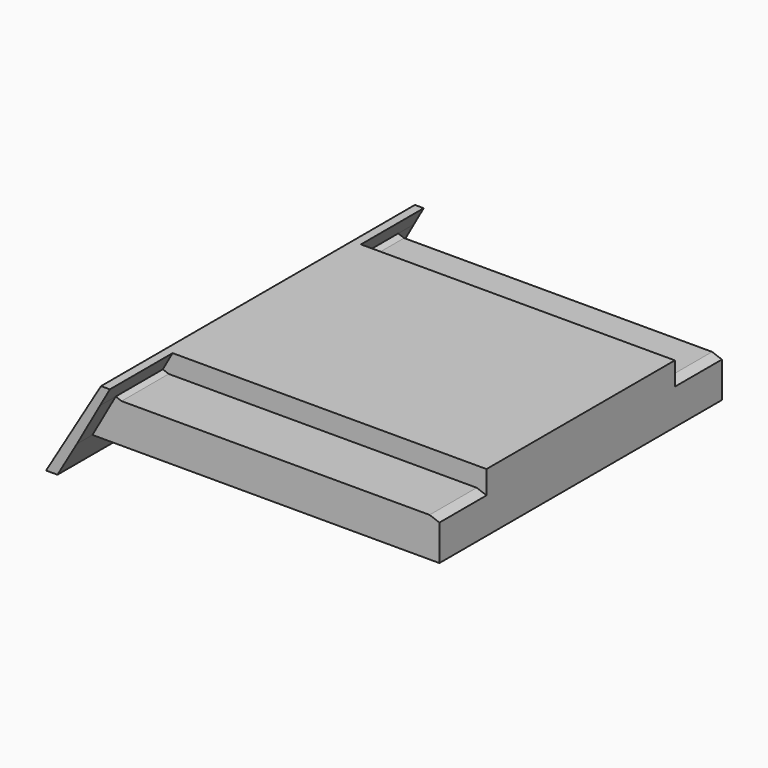
from build123d import *

# Parameters (mm, degrees)
F1_DEPTH  = 20
F3_DEPTH  = 4
F5_DEPTH  = 1
F7_DEPTH  = 20.001
F10_W     = 15
F10_H     = 9.1
F11_DEPTH = 1


# Not quite as in the source:
# - a pattern or mirror of a feature is missing from the dataset's text; its kind, count and spacing are read off the source's solid


with BuildPart() as f1:
    # F0 (on Front) → F1 (new body)
    with BuildSketch(Plane.XZ):
        Polygon((-16.45, 3), (-19.25, -1.7), (-18.09, -1.7), (-17.0772340426, 0), (0, 0), (0, 3), align=None)
    extrude(amount=F1_DEPTH)

    # F2 (on face) → F3 (cut)
    with BuildSketch(Plane.XZ.offset(20)):
        Polygon((-16.2, 2), (-0.5, 2), (0, 1.8180148829), (0, 3), (-16, 3), (-16.5, 2.1091910703), align=None)
    f3 = extrude(amount=-F3_DEPTH, mode=Mode.SUBTRACT)

    # F3_copies: F3 across plane
    add(f3.mirror(Plane.ZX.offset(-10)), mode=Mode.SUBTRACT)

    # F4 (on face) → F5 (cut)
    with BuildSketch(Plane.XZ.offset(20)):
        Polygon((0, 0), (0, 1.8180148829), (-0.5, 2), (-16.2, 2), (-16.5, 2.1091910703), (-17.683862779, 0), align=None)
    f5 = extrude(amount=-F5_DEPTH, mode=Mode.SUBTRACT)

    # F5_copies: F5 across plane
    add(f5.mirror(Plane.ZX.offset(-10)), mode=Mode.SUBTRACT)

    # F6 (on face) → F7 (cut, through all)
    with BuildSketch(Plane.XZ.offset(20)):
        Polygon((-18.67, -1.7), (-18.09, -1.7), (-17.0772340426, 0), (-17.683862779, 0), align=None)
    extrude(amount=-F7_DEPTH, mode=Mode.SUBTRACT)

    # F10 (on face) → F11 (cut)
    with BuildSketch(Plane(origin=(0, 0, 0), x_dir=(1, 0, 0), z_dir=(0, 0, -1))):
        with Locations((-9, 10)):
            Rectangle(F10_W, F10_H)
    extrude(amount=-F11_DEPTH, mode=Mode.SUBTRACT)


solid = f1.part
